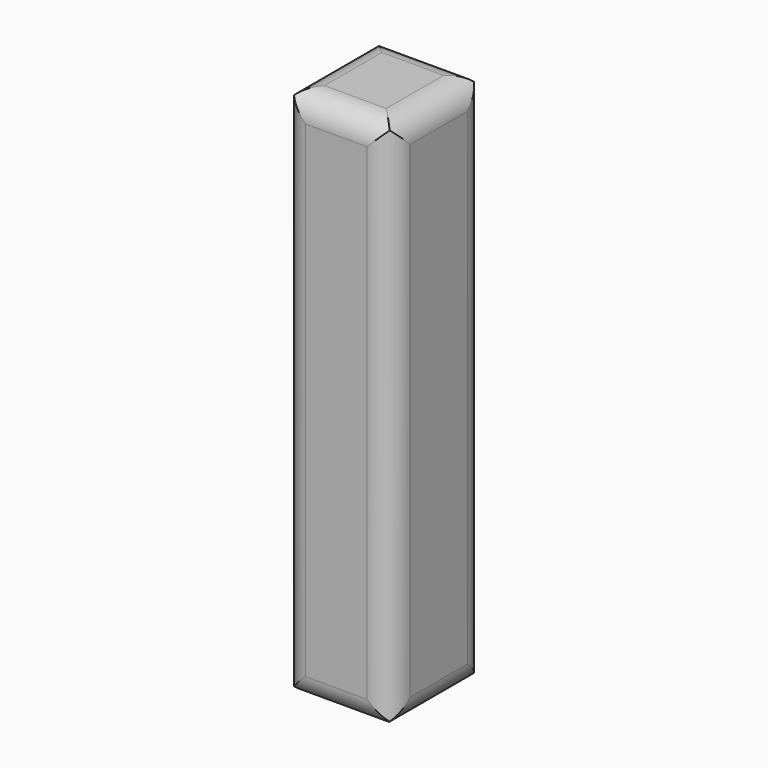
from build123d import *

# Parameters (mm, degrees)
F0_W        = 23.3076866716
F0_H        = 113.6004934087
F1_DEPTH    = 25.4
F2_R        = 5.08
F3_T1_DEPTH = 45.72
F3_T3_DEPTH = 139.0004934087
F4_T1_DEPTH = 45.72
F4_T3_DEPTH = 139.0004934087
F5_T1_DEPTH = 38.5476866716


# Not quite as in the source:
# - a fillet or chamfer that OpenCascade refuses, or shapes differently, is made with other operations: its cross-section is extruded or revolved along the edge and cut away or added


with BuildPart() as f1:
    # F0 (on Front) → F1 (new body)
    with BuildSketch(Plane.XZ):
        with Locations((0, -1.4689718373)):
            Rectangle(F0_W, F0_H)
    extrude(amount=F1_DEPTH)

    # F2
    f2_edges = [f1.edges().sort_by_distance(p)[0] for p in [
        (0, -25.4, 55.331275),
        (-11.653843, -25.4, -1.468972),
        (0, -25.4, -58.269219),
        (11.653843, -25.4, -1.468972),
    ]]
    fillet(f2_edges, radius=F2_R)

    # F3: fillet of radius 5.08 on 4 edges, made by hand

    # F3_s2 → F3_t1 (cut)
    with BuildSketch(Plane.XZ.offset(-12.7)):
        with BuildLine():
            ThreePointArc((11.6538433358, -53.1892185417), (10.1659457842, -56.7813209901), (6.5738433358, -58.2692185417))
            Line((6.5738433358, -58.2692185417), (11.6538433358, -58.2692185417))
            Line((11.6538433358, -58.2692185417), (11.6538433358, -53.1892185417))
        make_face()
        with BuildLine():
            ThreePointArc((6.5738433358, 55.3312748671), (10.1659457842, 53.8433773155), (11.6538433358, 50.2512748671))
            Line((11.6538433358, 50.2512748671), (11.6538433358, 55.3312748671))
            Line((11.6538433358, 55.3312748671), (6.5738433358, 55.3312748671))
        make_face()
    extrude(amount=F3_T1_DEPTH, mode=Mode.SUBTRACT)

    # F3_s4 → F3_t3 (cut)
    with BuildSketch(Plane.XY.offset(-70.9692185417)):
        with BuildLine():
            ThreePointArc((11.6538433358, -5.08), (10.1659457842, -1.4878975516), (6.5738433358, 0))
            Line((6.5738433358, 0), (11.6538433358, 0))
            Line((11.6538433358, 0), (11.6538433358, -5.08))
        make_face()
    extrude(amount=F3_T3_DEPTH, mode=Mode.SUBTRACT)

    # F4: fillet of radius 5.08 on 4 edges, made by hand

    # F4_s2 → F4_t1 (cut)
    with BuildSketch(Plane.XZ.offset(-12.7)):
        with BuildLine():
            ThreePointArc((-6.5738433358, 55.3312748671), (-10.1659457842, 53.8433773155), (-11.6538433358, 50.2512748671))
            Line((-11.6538433358, 50.2512748671), (-11.6538433358, 55.3312748671))
            Line((-11.6538433358, 55.3312748671), (-6.5738433358, 55.3312748671))
        make_face()
        with BuildLine():
            ThreePointArc((-11.6538433358, -53.1892185417), (-10.1659457842, -56.7813209901), (-6.5738433358, -58.2692185417))
            Line((-6.5738433358, -58.2692185417), (-11.6538433358, -58.2692185417))
            Line((-11.6538433358, -58.2692185417), (-11.6538433358, -53.1892185417))
        make_face()
    extrude(amount=F4_T1_DEPTH, mode=Mode.SUBTRACT)

    # F4_s4 → F4_t3 (cut)
    with BuildSketch(Plane.XY.offset(-70.9692185417)):
        with BuildLine():
            ThreePointArc((-6.5738433358, 0), (-10.1659457842, -1.4878975516), (-11.6538433358, -5.08))
            Line((-11.6538433358, -5.08), (-11.6538433358, 0))
            Line((-11.6538433358, 0), (-6.5738433358, 0))
        make_face()
    extrude(amount=F4_T3_DEPTH, mode=Mode.SUBTRACT)

    # F5: fillet of radius 5.08 on 4 edges, made by hand

    # F5_s2 → F5_t1 (cut)
    with BuildSketch(Plane.YZ.offset(-19.2738433358)):
        with BuildLine():
            ThreePointArc((-5.08, 55.3312748671), (-1.4878975516, 53.8433773155), (0, 50.2512748671))
            Line((0, 50.2512748671), (0, 55.3312748671))
            Line((0, 55.3312748671), (-5.08, 55.3312748671))
        make_face()
        with BuildLine():
            ThreePointArc((0, -53.1892185417), (-1.4878975516, -56.7813209901), (-5.08, -58.2692185417))
            Line((-5.08, -58.2692185417), (0, -58.2692185417))
            Line((0, -58.2692185417), (0, -53.1892185417))
        make_face()
    extrude(amount=F5_T1_DEPTH, mode=Mode.SUBTRACT)


solid = f1.part
